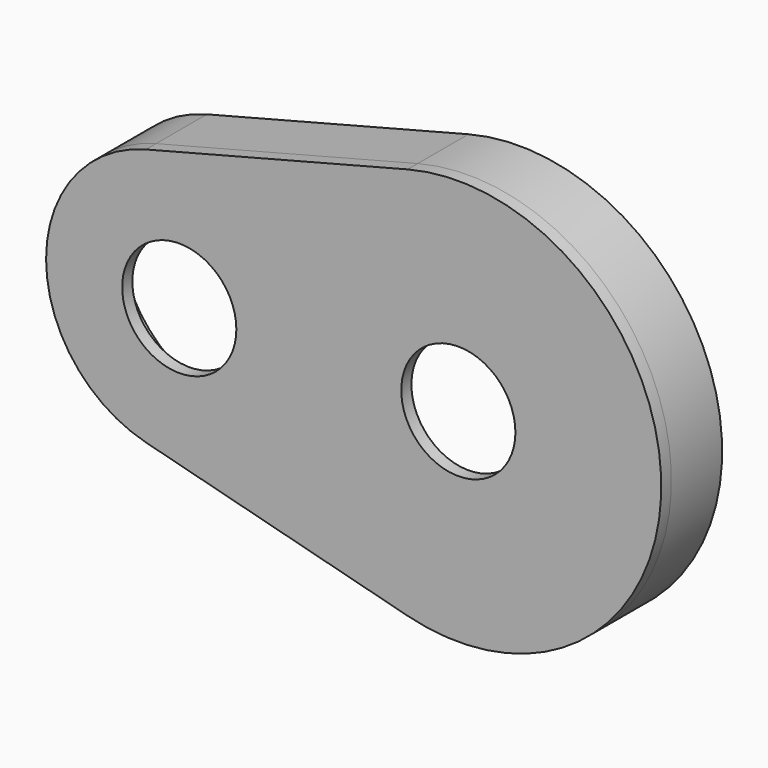
from build123d import *
from build123d import SkipClean  # not in build123d's __all__

# Parameters (mm, degrees)
F0_R     = 14.2875
F1_DEPTH = 3.175
F3_DEPTH = 15.875


with BuildPart() as f1:
    # F0 (on Front) → F1 (new body)
    with BuildSketch(Plane.XZ):
        with BuildLine():
            Line((-78.184375, -32.278895576), (-12.7, -49.1868884968))
            ThreePointArc((-12.7, -49.1868884968), (50.8, 0), (-12.7, 49.1868884968))
            Line((-12.7, 49.1868884968), (-78.184375, 32.278895576))
            ThreePointArc((-78.184375, 32.278895576), (-103.1875, 0), (-78.184375, -32.278895576))
        make_face()
        with Locations((-69.85, 0)):
            Circle(F0_R, mode=Mode.SUBTRACT)
        with BuildLine():
            ThreePointArc((-14.2875, 0), (0, 14.2875), (14.2875, 0))
            ThreePointArc((14.2875, 0), (0, -14.2875), (-14.2875, 0))
        make_face(mode=Mode.SUBTRACT)
    extrude(amount=F1_DEPTH)

    # F2 (on face) → F3 (join)
    with BuildSketch(Plane(origin=(0, 0, 0), x_dir=(-1, 0, 0), z_dir=(0, 1, 0))):
        with BuildLine():
            ThreePointArc((78.184375, -32.278895576), (103.1875, 0), (78.184375, 32.278895576))
            Line((78.184375, 32.278895576), (12.7, 49.1868884968))
            ThreePointArc((12.7, 49.1868884968), (-50.8, 0), (12.7, -49.1868884968))
            Line((12.7, -49.1868884968), (78.184375, -32.278895576))
        make_face()
        with BuildLine():
            Line((11.90625, 46.1127079658), (77.390625, 29.204715045))
            ThreePointArc((77.390625, 29.204715045), (100.0125, 0), (77.390625, -29.204715045))
            Line((77.390625, -29.204715045), (11.90625, -46.1127079658))
            ThreePointArc((11.90625, -46.1127079658), (-47.625, 0), (11.90625, 46.1127079658))
        make_face(mode=Mode.SUBTRACT)
    with SkipClean():  # cleaning this boolean's faces spoils the solid; the shape is the same uncleaned
        extrude(amount=F3_DEPTH)


solid = f1.part
